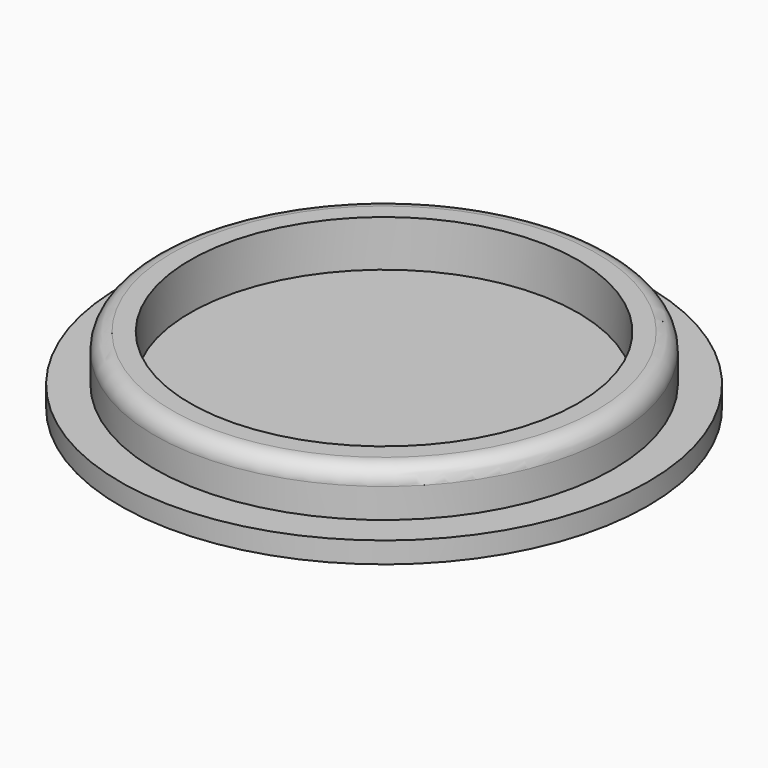
from build123d import *

# Parameters (mm, degrees)
F0_R     = 39.751
F0_R_2   = 34.544
F1_DEPTH = 3.175
F0_R_3   = 29.21
F2_DEPTH = 10.16
F3_R     = 2.54


with BuildPart() as f1:
    # F0 (on Top) → F1 (new body)
    with BuildSketch(Plane.XY):
        Circle(F0_R)
        Circle(F0_R_2, mode=Mode.SUBTRACT)
    extrude(amount=F1_DEPTH)

    # F0 (on Top) → F2 (join)
    with BuildSketch(Plane.XY):
        Circle(F0_R_2)
        Circle(F0_R_3, mode=Mode.SUBTRACT)
    extrude(amount=F2_DEPTH)

    # F3
    f3_edges = [f1.edges().sort_by_distance(p)[0] for p in [
        (-34.544, 0, 10.16),
    ]]
    fillet(f3_edges, radius=F3_R)


with BuildPart() as f1b:
    # F0 (on Top) → F1, piece 2 (new body)
    with BuildSketch(Plane.XY):
        Circle(F0_R_3)
    extrude(amount=F1_DEPTH)


solid = Compound([f1.part, f1b.part])
